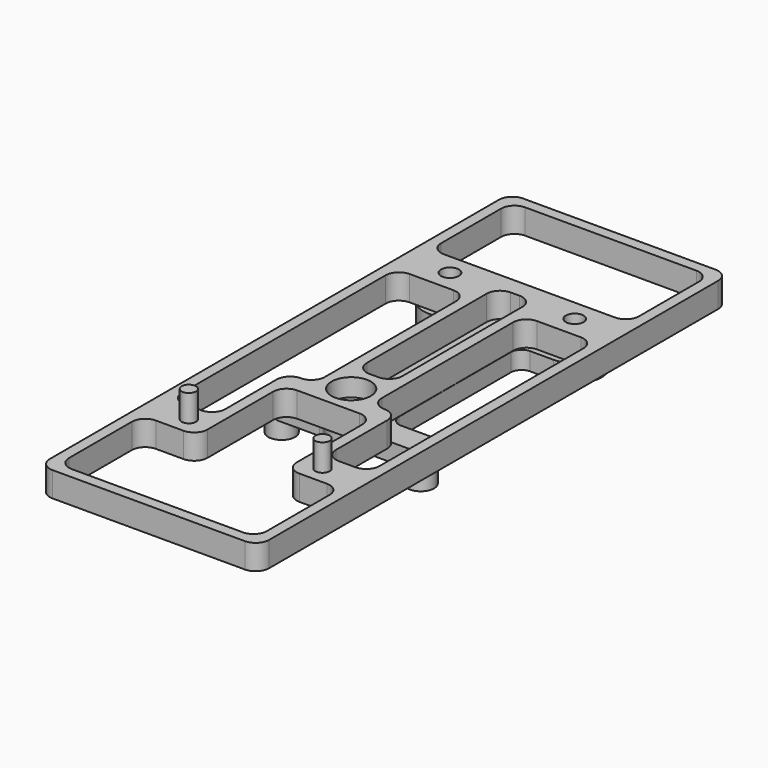
from build123d import *

# Parameters (mm, degrees)
F0_W      = 31.242
F0_H      = 83.82
F0_R      = 1.524
F0_R_2    = 1.27
F0_W_2    = 5.08
F0_H_2    = 25.146
F0_W_3    = 28.194
F0_H_3    = 14.478
F1_DEPTH  = 3.556
F2_R      = 1.90499
F3_R      = 1.016
F4_DEPTH  = 3.81
F5_R      = 2.794
F6_DEPTH  = 2.54
F8_R      = 1.524
F8_R_2    = 1.27
F9_DEPTH  = 2.54
F10_R     = 1.524
F11_R     = 1.905
F12_DEPTH = 2.54


# Not quite as in the source:
# - a fillet or chamfer is up to 0.001 mm smaller than in the source, because OpenCascade refuses the exact size
# - after a boolean that leaves OpenCascade's solid faulty, fix() repairs it


with BuildPart() as f1:
    # F0 (on Top) → F1 (new body)
    with BuildSketch(Plane.XY):
        Rectangle(F0_W, F0_H)
        Polygon((-14.097, -20.32), (-14.097, 19.812), (-4.064, 19.812), (-4.064, -7.366), (-7.874, -7.366), (-7.874, -20.32), align=None, mode=Mode.SUBTRACT)
        Polygon((14.097, -40.386), (-14.097, -40.386), (-14.097, -25.4), (-6.35, -25.4), (-6.35, -9.906), (6.35, -9.906), (6.35, -25.4), (14.097, -25.4), align=None, mode=Mode.SUBTRACT)
        with Locations((0, -5.842)):
            Circle(F0_R, mode=Mode.SUBTRACT)
        Polygon((4.064, 19.812), (14.097, 19.812), (14.097, -20.32), (7.874, -20.32), (7.874, -7.366), (4.064, -7.366), align=None, mode=Mode.SUBTRACT)
        with Locations((-8.89, 22.86)):
            Circle(F0_R_2, mode=Mode.SUBTRACT)
        with Locations((0, 10.795)):
            Rectangle(F0_W_2, F0_H_2, mode=Mode.SUBTRACT)
        with Locations((0, 33.147)):
            Rectangle(F0_W_3, F0_H_3, mode=Mode.SUBTRACT)
        with Locations((8.89, 22.86)):
            Circle(F0_R_2, mode=Mode.SUBTRACT)
    extrude(amount=F1_DEPTH)

    # F2 (radius 1.905 in the source; OpenCascade refuses exactly that, so slightly less here)
    f2_edges = [f1.edges().sort_by_distance(p)[0] for p in [
        (14.097, 40.386, 1.778),
        (-14.097, 40.386, 1.778),
        (-14.097, 25.908, 1.778),
        (14.097, 25.908, 1.778),
        (-15.621, 41.91, 1.778),
        (15.621, 41.91, 1.778),
        (-2.54, 23.368, 1.778),
        (-14.097, 19.812, 1.778),
        (4.064, 19.812, 1.778),
        (-4.064, 19.812, 1.778),
        (2.54, 23.368, 1.778),
        (14.097, 19.812, 1.778),
        (-7.874, -20.32, 1.778),
        (-7.874, -7.366, 1.778),
        (-4.064, -7.366, 1.778),
        (2.54, -1.778, 1.778),
        (7.874, -7.366, 1.778),
        (14.097, -20.32, 1.778),
        (14.097, -40.386, 1.778),
        (6.35, -25.4, 1.778),
        (-14.097, -20.32, 1.778),
        (7.874, -20.32, 1.778),
        (4.064, -7.366, 1.778),
        (-2.54, -1.778, 1.778),
        (-6.35, -25.4, 1.778),
        (-14.097, -40.386, 1.778),
        (-14.097, -25.4, 1.778),
        (-6.35, -9.906, 1.778),
        (14.097, -25.4, 1.778),
        (6.35, -9.906, 1.778),
        (-15.621, -41.91, 1.778),
        (15.621, -41.91, 1.778),
    ]]
    fillet(f2_edges, radius=F2_R)

    # F3 (on face) → F4 (join)
    with BuildSketch(Plane.XY.offset(3.556)):
        with Locations((-9.525, -22.86)):
            Circle(F3_R)
        with Locations((9.525, -22.86)):
            Circle(F3_R)
    extrude(amount=F4_DEPTH)

    # F5 (on face) → F6 (cut)
    with BuildSketch(Plane.XY.offset(3.556)):
        with Locations((0, -5.842)):
            Circle(F5_R)
    extrude(amount=-F6_DEPTH, mode=Mode.SUBTRACT)


with BuildPart() as f9:
    # F8 (on offset) → F9 (new body)
    with BuildSketch(Plane.XY.offset(-0.0254)):
        with BuildLine():
            Line((2.3793442374, -7.747), (9.906, -7.747))
            ThreePointArc((9.906, -7.747), (11.811, -5.842), (9.906, -3.937))
            Line((9.906, -3.937), (4.064, -3.937))
            Line((4.064, -3.937), (4.064, 19.05))
            Line((4.064, 19.05), (8.89, 19.05))
            ThreePointArc((8.89, 19.05), (12.7, 22.86), (8.89, 26.67))
            Line((8.89, 26.67), (-8.89, 26.67))
            ThreePointArc((-8.89, 26.67), (-12.7, 22.86), (-8.89, 19.05))
            Line((-8.89, 19.05), (-4.064, 19.05))
            Line((-4.064, 19.05), (-4.064, -3.937))
            Line((-4.064, -3.937), (-9.906, -3.937))
            ThreePointArc((-9.906, -3.937), (-11.811, -5.842), (-9.906, -7.747))
            Line((-9.906, -7.747), (-2.3793442374, -7.747))
            ThreePointArc((-2.3793442374, -7.747), (0, -8.89), (2.3793442374, -7.747))
        make_face()
        with Locations((0, -5.842)):
            Circle(F8_R, mode=Mode.SUBTRACT)
        with Locations((-8.89, 22.86)):
            Circle(F8_R_2, mode=Mode.SUBTRACT)
        with Locations((8.89, 22.86)):
            Circle(F8_R_2, mode=Mode.SUBTRACT)
    extrude(amount=-F9_DEPTH)

    # F10
    f10_edges = [f9.edges().sort_by_distance(p)[0] for p in [
        (-4.064, -3.937, -1.2954),
        (4.064, -3.937, -1.2954),
        (2.379344, -7.747, -1.2954),
        (-2.379344, -7.747, -1.2954),
        (-4.064, 19.05, -1.2954),
        (4.064, 19.05, -1.2954),
    ]]
    fillet(f10_edges, radius=F10_R)

    # F11 (on face) → F12 (join)
    with BuildSketch(Plane(origin=(0, 0, -2.5654), x_dir=(1, 0, 0), z_dir=(0, 0, -1))):
        with Locations((9.906, 5.842)):
            Circle(F11_R)
        with Locations((-9.906, 5.842)):
            Circle(F11_R)
    extrude(amount=F12_DEPTH)

    add(f9.part.fix(), mode=Mode.REPLACE)


solid = Compound([f1.part, f9.part])
